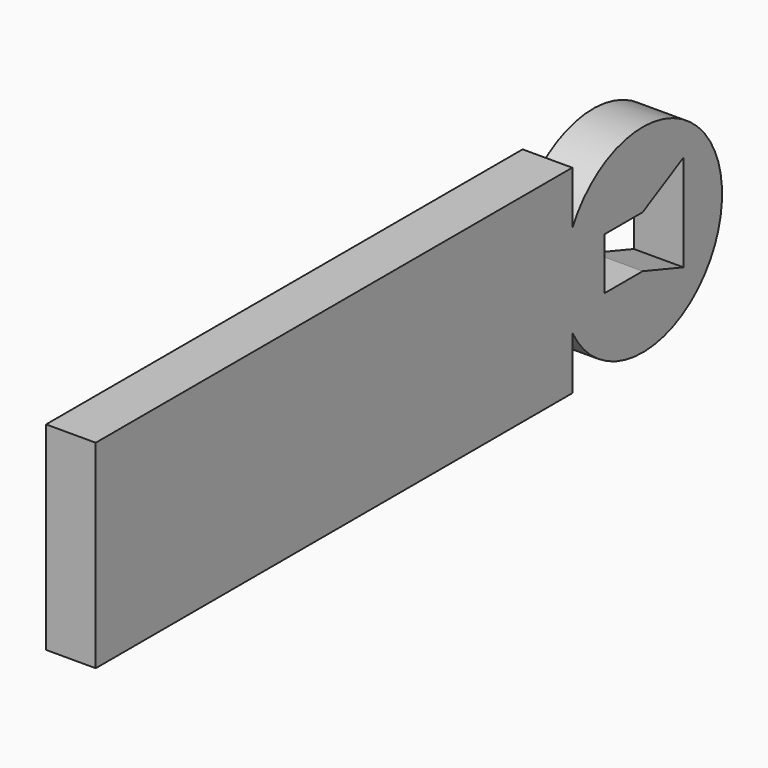
from build123d import *

# Parameters (mm, degrees)
F1_DEPTH = 12.7


# Not quite as in the source:
# - the program builds the solid bodies; features that only make, move or delete a surface that nothing else refers to are left out


with BuildPart() as f1:
    # F0 (on Right) → F1 (new body)
    with BuildSketch(Plane.YZ):
        with BuildLine():
            Line((-22.5137730746, 11.7596777994), (-22.5137730746, 25.4))
            Line((-22.5137730746, 25.4), (-174.9137730746, 25.4))
            Line((-174.9137730746, 25.4), (-174.9137730746, -25.4))
            Line((-174.9137730746, -25.4), (-22.5137730746, -25.4))
            Line((-22.5137730746, -25.4), (-22.5137730746, -11.7596777994))
            ThreePointArc((-22.5137730746, -11.7596777994), (25.4, 0), (-22.5137730746, 11.7596777994))
        make_face()
        Polygon((-12.2498031706, -7.0739961229), (-12.2498031706, 6.2070912682), (0, 6.2070912682), (13.0541240796, 13.2165625691), (13.0541240796, -11.5010300651), (0, -7.0739961229), align=None, mode=Mode.SUBTRACT)
    extrude(amount=F1_DEPTH)


solid = f1.part
